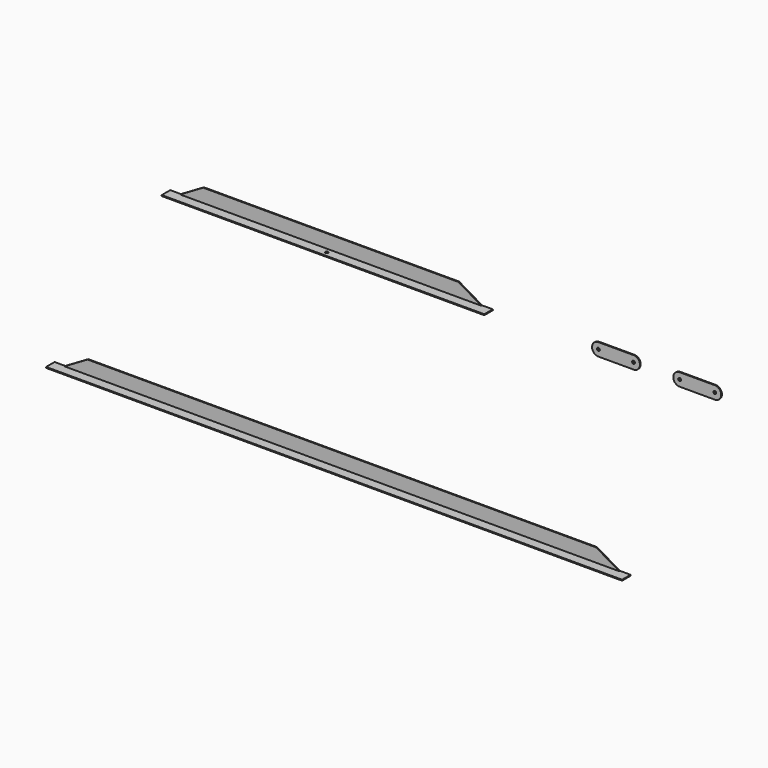
from build123d import *

# Parameters (mm, degrees)
F1_DEPTH = 11.7348
F2_R     = 1.5875
F3_DEPTH = 1.016
F4_T     = 1.016
F5_T     = 1.016
F6_R     = 1.5875
F7_DEPTH = 228.6


# Not quite as in the source:
# - a shell that OpenCascade refuses in one call is made with other operations: the cavity is built on its own and cut out


with BuildPart() as f1:
    # F0 (on Front) → F1 (new body)
    with BuildSketch(Plane.XZ):
        Polygon((-385.423819233, -32.3961665051), (-373.689019233, -32.3961665051), (237.841380767, -32.3961665051), (249.576180767, -32.3961665051), (249.576180767, -31.3801665051), (237.841380767, -31.3801665051), (212.441380767, -16.5211665051), (-348.289019233, -16.5211665051), (-373.689019233, -31.3801665051), (-385.423819233, -31.3801665051), align=None)
    extrude(amount=F1_DEPTH)

    # F4: shell of thickness 1.016, made by hand


with BuildPart() as f1b:
    # F0 (on Front) → F1, piece 2 (new body)
    with BuildSketch(Plane.XZ):
        Polygon((-257.9213991354, 175.8537739515), (-246.1865991354, 175.8537739515), (85.9438008646, 175.8537739515), (97.6786008646, 175.8537739515), (97.6786008646, 176.8697739515), (85.9438008646, 176.8697739515), (60.5438008646, 191.7287739515), (-220.7865991354, 191.7287739515), (-246.1865991354, 176.8697739515), (-257.9213991354, 176.8697739515), align=None)
    extrude(amount=F1_DEPTH)

    # F5: shell of thickness 1.016, made by hand


with BuildPart() as f3:
    # F2 (on Front) → F3 (new body)
    with BuildSketch(Plane.XZ):
        with BuildLine():
            Line((253.6772660458, 183.5175923166), (214.8952760458, 183.5175923166))
            ThreePointArc((214.8952760458, 183.5175923166), (207.888375372, 176.5106916428), (214.8952760458, 169.503790969))
            Line((214.8952760458, 169.503790969), (253.6772660458, 169.503790969))
            ThreePointArc((253.6772660458, 169.503790969), (260.6841667196, 176.5106916428), (253.6772660458, 183.5175923166))
        make_face()
        with Locations((214.8952760458, 176.5106916428)):
            Circle(F2_R, mode=Mode.SUBTRACT)
        with Locations((253.6772660458, 176.5106916428)):
            Circle(F2_R, mode=Mode.SUBTRACT)
    extrude(amount=F3_DEPTH)


with BuildPart() as f3b:
    # F2 (on Front) → F3, piece 2 (new body)
    with BuildSketch(Plane.XZ):
        with BuildLine():
            Line((343.2592560458, 183.4247431812), (304.4772660458, 183.4247431812))
            ThreePointArc((304.4772660458, 183.4247431812), (297.470365372, 176.4178425074), (304.4772660458, 169.4109418336))
            Line((304.4772660458, 169.4109418336), (343.2592560458, 169.4109418336))
            ThreePointArc((343.2592560458, 169.4109418336), (350.2661567196, 176.4178425074), (343.2592560458, 183.4247431812))
        make_face()
        with Locations((304.4772660458, 176.4178425074)):
            Circle(F2_R, mode=Mode.SUBTRACT)
        with Locations((343.2592560458, 176.4178425074)):
            Circle(F2_R, mode=Mode.SUBTRACT)
    extrude(amount=F3_DEPTH)


with BuildPart() as f4_core1:
    # F4_t2: copy of F1
    add(f1.part)

    # the walls: a layer under each face that stays
    f4_faces = [f4_core1.faces().sort_by_distance(p)[0] for p in [
        (-67.923819233, -5.8674, -32.3961665051),
        (-67.923819233, 0, -24.4586665051),
        (-379.556419233, -5.8674, -31.3801665051),
        (243.708780767, -5.8674, -31.3801665051),
        (249.576180767, -5.8674, -31.8881665051),
        (-385.423819233, -5.8674, -31.8881665051),
    ]]
    thicken(f4_faces, amount=-F4_T, mode=Mode.SUBTRACT)


with BuildPart() as f1_1:
    add(f1.part)

    # what is left inside the walls is the cavity
    f4_cavity = [f4_core1.part.solids().sort_by_distance(p)[0] for p in [
        (-67.923819, -1.02616, -26.427167),
    ]]
    add(f4_cavity, mode=Mode.SUBTRACT)


with BuildPart() as f5_core1:
    # F5_t2: copy of F1b
    add(f1b.part)

    # the walls: a layer under each face that stays
    f5_faces = [f5_core1.faces().sort_by_distance(p)[0] for p in [
        (-80.1213991354, -5.8674, 175.8537739515),
        (-80.1213991354, 0, 183.7912739515),
        (-252.0539991354, -5.8674, 176.8697739515),
        (91.8112008646, -5.8674, 176.8697739515),
        (97.6786008646, -5.8674, 176.3617739515),
        (-257.9213991354, -5.8674, 176.3617739515),
    ]]
    thicken(f5_faces, amount=-F5_T, mode=Mode.SUBTRACT)


with BuildPart() as f1b_1:
    add(f1b.part)

    # what is left inside the walls is the cavity
    f5_cavity = [f5_core1.part.solids().sort_by_distance(p)[0] for p in [
        (-80.121399, -1.02616, 181.822774),
    ]]
    add(f5_cavity, mode=Mode.SUBTRACT)

    # F6 (on Top) → F7 (cut)
    with BuildSketch(Plane.XY):
        with Locations((-80.1213991354, -6.3754)):
            Circle(F6_R)
    extrude(amount=F7_DEPTH, mode=Mode.SUBTRACT)


solid = Compound([f3.part, f3b.part, f1_1.part, f1b_1.part])
